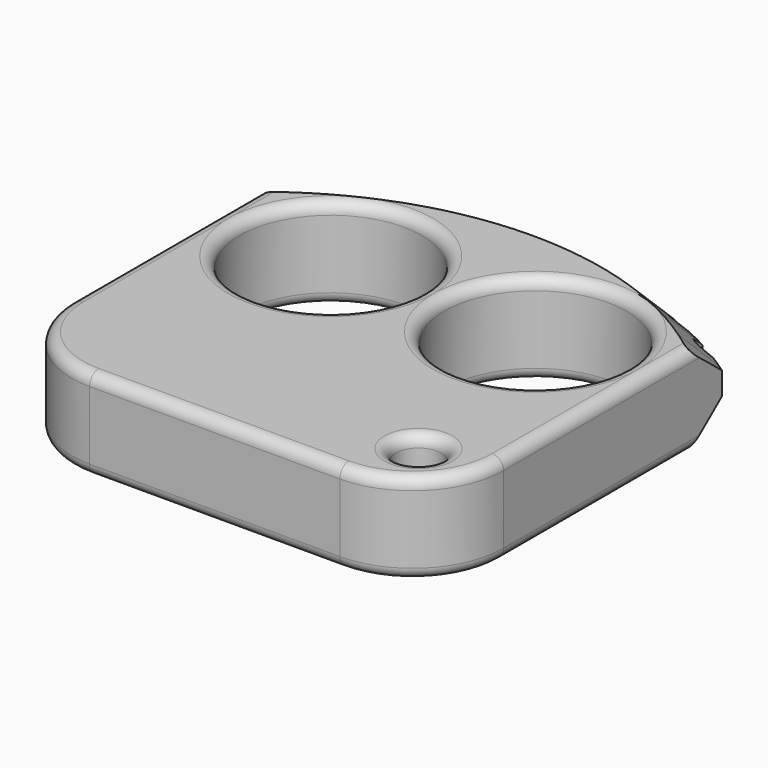
from build123d import *

# Parameters (mm, degrees)
F0_R         = 3.175
F0_R_2       = 12.7
F1_DEPTH     = 12.7
F2_R         = 1.58749
F3_T2_ANGLE  = 28.2217066526
F3_T4_ANGLE  = 30.4023138014
F3_T6_ANGLE  = 28.2217066526
F3_T8_ANGLE  = 30.7280198059
F3_T10_ANGLE = 30.527086938
F3_T12_ANGLE = 28.2217066526
F3_T14_ANGLE = 30.7280198059
F3_T16_ANGLE = 31.8182338751
F3_T18_ANGLE = 30.3249155811
F3_T20_ANGLE = 32.0978046052
F3_T22_ANGLE = 30.3249155811
F3_T24_ANGLE = 30.7280198059
F3_T26_ANGLE = 30.527086938
F3_T28_ANGLE = 28.2217066526
F3_T30_ANGLE = 30.4023138014
F3_T32_ANGLE = 30.7280198059
F3_T34_ANGLE = 31.8182338751
F3_T36_ANGLE = 30.3249155811
F3_T38_ANGLE = 32.0978046052
F3_T40_ANGLE = 30.3249155811
F4_DEPTH     = 25.4
F5_R         = 1.5875


# Not quite as in the source:
# - a fillet or chamfer that OpenCascade refuses, or shapes differently, is made with other operations: its cross-section is extruded or revolved along the edge and cut away or added
# - a fillet or chamfer is up to 0.001 mm smaller than in the source, because OpenCascade refuses the exact size


with BuildPart() as f1:
    # F0 (on Top) → F1 (new body)
    with BuildSketch(Plane.XY):
        with BuildLine():
            Line((30.1625, -25.4), (30.1625, 12.7))
            ThreePointArc((30.1625, 12.7), (28.8519314022, 13.5961848997), (27.5147547248, 14.4521615101))
            ThreePointArc((27.5147547248, 14.4521615101), (25.3582525776, 13.8924409049), (24.7658556955, 16.0401966174))
            ThreePointArc((24.7658556955, 16.0401966174), (23.1916703305, 16.8528451099), (21.5908556955, 17.6116926836))
            ThreePointArc((21.5908556955, 17.6116926836), (19.5238646988, 16.7802259757), (18.6611120255, 18.8343551079))
            ThreePointArc((18.6611120255, 18.8343551079), (17.1695789211, 19.3784749682), (15.6622115379, 19.8770539453))
            ThreePointArc((15.6622115379, 19.8770539453), (13.7112016409, 18.8012523611), (12.6059031197, 20.7357041816))
            ThreePointArc((12.6059031197, 20.7357041816), (11.059428231, 21.095082593), (9.5027540199, 21.4073370162))
            ThreePointArc((9.5027540199, 21.4073370162), (7.6964771744, 20.103054599), (6.3649215437, 21.8893211718))
            ThreePointArc((6.3649215437, 21.8893211718), (3.980300573, 22.1264782009), (1.5873170269, 22.2541119659))
            ThreePointArc((1.5873170269, 22.2541119659), (0, 20.6907139607), (-1.5873170269, 22.2541119659))
            ThreePointArc((-1.5873170269, 22.2541119659), (-3.8531098679, 22.1360337195), (-6.1116459836, 21.9197600851))
            ThreePointArc((-6.1116459836, 21.9197600851), (-7.4519015724, 20.1400118941), (-9.2517928734, 21.4530922311))
            ThreePointArc((-9.2517928734, 21.4530922311), (-10.8445183187, 21.1411241295), (-12.4267928734, 20.7798684392))
            ThreePointArc((-12.4267928734, 20.7798684392), (-13.5389102559, 18.8493287233), (-15.4861120255, 19.9320077778))
            ThreePointArc((-15.4861120255, 19.9320077778), (-17.0824306802, 19.4086897201), (-18.6611120255, 18.8343551079))
            ThreePointArc((-18.6611120255, 18.8343551079), (-19.5238646988, 16.7802259757), (-21.5908556955, 17.6116926836))
            ThreePointArc((-21.5908556955, 17.6116926836), (-23.1916703305, 16.8528451099), (-24.7658556955, 16.0401966174))
            ThreePointArc((-24.7658556955, 16.0401966174), (-25.3582525776, 13.8924409049), (-27.5147547248, 14.4521615101))
            ThreePointArc((-27.5147547248, 14.4521615101), (-28.8519314022, 13.5961848997), (-30.1625, 12.7))
            Line((-30.1625, 12.7), (-30.1625, -25.4))
            ThreePointArc((-30.1625, -25.4), (-26.4427561211, -34.3802561211), (-17.4625, -38.1))
            Line((-17.4625, -38.1), (17.4625, -38.1))
            ThreePointArc((17.4625, -38.1), (26.4427561211, -34.3802561211), (30.1625, -25.4))
        make_face()
        with Locations((21.5674359697, -29.5049359697)):
            Circle(F0_R, mode=Mode.SUBTRACT)
        with Locations((-14.2875, 0)):
            Circle(F0_R_2, mode=Mode.SUBTRACT)
        with Locations((14.2875, 0)):
            Circle(F0_R_2, mode=Mode.SUBTRACT)
    extrude(amount=F1_DEPTH)

    # F2 (radius 1.5875 in the source; OpenCascade refuses exactly that, so slightly less here)
    f2_edges = [f1.edges().sort_by_distance(p)[0] for p in [
        (0, -38.1, 12.7),
        (0, -38.1, 0),
        (-1.5875, 0, 6.35),
        (-26.9875, 0, 0),
        (-26.9875, 0, 12.7),
        (26.9875, 0, 6.35),
        (1.5875, 0, 0),
        (1.5875, 0, 12.7),
    ]]
    fillet(f2_edges, radius=F2_R)

    # F3: chamfer of 4.7625 on 20 edges, made by hand

    # F3_s1 → F3_t2 (revolve, cut)
    with BuildSketch(Plane(origin=(-8.957835853, -2.9681397895, 0), x_dir=(0, 0, 1), z_dir=(0.9492478243, 0.3145291211, 0))):
        Polygon((7.9375, -23.8009242864), (12.7, -19.0384242864), (12.7, -23.8009242864), align=None)
    revolve(axis=Axis((0, -30.0028581179, 12.7), (0, 0, 1)), revolution_arc=F3_T2_ANGLE, mode=Mode.SUBTRACT)

    # F3_s3 → F3_t4 (revolve, cut)
    with BuildSketch(Plane(origin=(1.6875607635, -0.0952218794, 0), x_dir=(0, 0, 1), z_dir=(0.9984118588, -0.0563361365, 0))):
        Polygon((0, -17.5633627369), (4.7625, -22.3258627369), (0, -22.3258627369), align=None)
    revolve(axis=Axis((0, -30.0028581179, 0), (0, 0, 1)), revolution_arc=F3_T4_ANGLE, mode=Mode.SUBTRACT)

    # F3_s5 → F3_t6 (revolve, cut)
    with BuildSketch(Plane(origin=(-8.957835853, -2.9681397895, 0), x_dir=(0, 0, 1), z_dir=(0.9492478243, 0.3145291211, 0))):
        Polygon((4.7625, -23.8009242864), (0, -19.0384242864), (0, -23.8009242864), align=None)
    revolve(axis=Axis((0, -30.0028581179, 0), (0, 0, 1)), revolution_arc=F3_T6_ANGLE, mode=Mode.SUBTRACT)

    # F3_s7 → F3_t8 (revolve, cut)
    with BuildSketch(Plane(origin=(-5.604837916, -1.0863772895, 0), x_dir=(0, 0, 1), z_dir=(0.9817285131, 0.1902869587, 0))):
        Polygon((0, -18.0639107911), (4.7625, -22.8264107911), (0, -22.8264107911), align=None)
    revolve(axis=Axis((0, -30.0028581179, 0), (0, 0, 1)), revolution_arc=F3_T8_ANGLE, mode=Mode.SUBTRACT)

    # F3_s9 → F3_t10 (revolve, cut)
    with BuildSketch(Plane(origin=(-1.9879865723, -0.1323072557, 0), x_dir=(0, 0, 1), z_dir=(0.9977926529, 0.0664064886, 0))):
        Polygon((0, -17.5819406812), (4.7625, -22.3444406812), (0, -22.3444406812), align=None)
    revolve(axis=Axis((0, -30.0028581179, 0), (0, 0, 1)), revolution_arc=F3_T10_ANGLE, mode=Mode.SUBTRACT)

    # F3_s11 → F3_t12 (revolve, cut)
    with BuildSketch(Plane(origin=(14.9793608703, -15.8148303911, 0), x_dir=(0, 0, 1), z_dir=(0.687669401, -0.726023963, 0))):
        Polygon((0, -26.8865246073), (4.7625, -31.6490246073), (0, -31.6490246073), align=None)
    revolve(axis=Axis((0, -30.0028581179, 0), (0, 0, 1)), revolution_arc=F3_T12_ANGLE, mode=Mode.SUBTRACT)

    # F3_s13 → F3_t14 (revolve, cut)
    with BuildSketch(Plane(origin=(14.9018636239, -13.275933668, 0), x_dir=(0, 0, 1), z_dir=(0.746666615, -0.6651984411, 0))):
        Polygon((0, -25.1164395681), (4.7625, -29.8789395681), (0, -29.8789395681), align=None)
    revolve(axis=Axis((0, -30.0028581179, 0), (0, 0, 1)), revolution_arc=F3_T14_ANGLE, mode=Mode.SUBTRACT)

    # F3_s15 → F3_t16 (revolve, cut)
    with BuildSketch(Plane(origin=(5.9494186304, -1.2301803221, 0), x_dir=(0, 0, 1), z_dir=(0.9792843793, -0.2024897638, 0))):
        Polygon((0, -18.1372417891), (4.7625, -22.8997417891), (0, -22.8997417891), align=None)
    revolve(axis=Axis((0, -30.0028581179, 0), (0, 0, 1)), revolution_arc=F3_T16_ANGLE, mode=Mode.SUBTRACT)

    # F3_s17 → F3_t18 (revolve, cut)
    with BuildSketch(Plane(origin=(13.9737874605, -9.5446774776, 0), x_dir=(0, 0, 1), z_dir=(0.8257568602, -0.5640262475, 0))):
        Polygon((0, -22.7435061634), (4.7625, -27.5060061634), (0, -27.5060061634), align=None)
    revolve(axis=Axis((0, -30.0028581179, 0), (0, 0, 1)), revolution_arc=F3_T18_ANGLE, mode=Mode.SUBTRACT)

    # F3_s19 → F3_t20 (revolve, cut)
    with BuildSketch(Plane(origin=(9.808271153, -3.6506277304, 0), x_dir=(0, 0, 1), z_dir=(0.9371894158, -0.3488208693, 0))):
        Polygon((0, -19.4002110061), (4.7625, -24.1627110061), (0, -24.1627110061), align=None)
    revolve(axis=Axis((0, -30.0028581179, 0), (0, 0, 1)), revolution_arc=F3_T20_ANGLE, mode=Mode.SUBTRACT)

    # F3_s21 → F3_t22 (revolve, cut)
    with BuildSketch(Plane(origin=(12.2507752992, -6.3434051286, 0), x_dir=(0, 0, 1), z_dir=(0.8880165005, -0.4598115863, 0))):
        Polygon((0, -20.8755390083), (4.7625, -25.6380390083), (0, -25.6380390083), align=None)
    revolve(axis=Axis((0, -30.0028581179, 0), (0, 0, 1)), revolution_arc=F3_T22_ANGLE, mode=Mode.SUBTRACT)

    # F3_s23 → F3_t24 (revolve, cut)
    with BuildSketch(Plane(origin=(-5.604837916, -1.0863772895, 0), x_dir=(0, 0, 1), z_dir=(0.9817285131, 0.1902869587, 0))):
        Polygon((12.7, -18.0639107911), (7.9375, -22.8264107911), (12.7, -22.8264107911), align=None)
    revolve(axis=Axis((0, -30.0028581179, 12.7), (0, 0, 1)), revolution_arc=F3_T24_ANGLE, mode=Mode.SUBTRACT)

    # F3_s25 → F3_t26 (revolve, cut)
    with BuildSketch(Plane(origin=(-1.9879865723, -0.1323072557, 0), x_dir=(0, 0, 1), z_dir=(0.9977926529, 0.0664064886, 0))):
        Polygon((12.7, -17.5819406812), (7.9375, -22.3444406812), (12.7, -22.3444406812), align=None)
    revolve(axis=Axis((0, -30.0028581179, 12.7), (0, 0, 1)), revolution_arc=F3_T26_ANGLE, mode=Mode.SUBTRACT)

    # F3_s27 → F3_t28 (revolve, cut)
    with BuildSketch(Plane(origin=(14.9793608703, -15.8148303911, 0), x_dir=(0, 0, 1), z_dir=(0.687669401, -0.726023963, 0))):
        Polygon((12.7, -26.8865246073), (7.9375, -31.6490246073), (12.7, -31.6490246073), align=None)
    revolve(axis=Axis((0, -30.0028581179, 12.7), (0, 0, 1)), revolution_arc=F3_T28_ANGLE, mode=Mode.SUBTRACT)

    # F3_s29 → F3_t30 (revolve, cut)
    with BuildSketch(Plane(origin=(1.6875607635, -0.0952218794, 0), x_dir=(0, 0, 1), z_dir=(0.9984118588, -0.0563361365, 0))):
        Polygon((12.7, -17.5633627369), (7.9375, -22.3258627369), (12.7, -22.3258627369), align=None)
    revolve(axis=Axis((0, -30.0028581179, 12.7), (0, 0, 1)), revolution_arc=F3_T30_ANGLE, mode=Mode.SUBTRACT)

    # F3_s31 → F3_t32 (revolve, cut)
    with BuildSketch(Plane(origin=(14.9018636239, -13.275933668, 0), x_dir=(0, 0, 1), z_dir=(0.746666615, -0.6651984411, 0))):
        Polygon((12.7, -25.1164395681), (7.9375, -29.8789395681), (12.7, -29.8789395681), align=None)
    revolve(axis=Axis((0, -30.0028581179, 12.7), (0, 0, 1)), revolution_arc=F3_T32_ANGLE, mode=Mode.SUBTRACT)

    # F3_s33 → F3_t34 (revolve, cut)
    with BuildSketch(Plane(origin=(5.9494186304, -1.2301803221, 0), x_dir=(0, 0, 1), z_dir=(0.9792843793, -0.2024897638, 0))):
        Polygon((12.7, -18.1372417891), (7.9375, -22.8997417891), (12.7, -22.8997417891), align=None)
    revolve(axis=Axis((0, -30.0028581179, 12.7), (0, 0, 1)), revolution_arc=F3_T34_ANGLE, mode=Mode.SUBTRACT)

    # F3_s35 → F3_t36 (revolve, cut)
    with BuildSketch(Plane(origin=(13.9737874605, -9.5446774776, 0), x_dir=(0, 0, 1), z_dir=(0.8257568602, -0.5640262475, 0))):
        Polygon((12.7, -22.7435061634), (7.9375, -27.5060061634), (12.7, -27.5060061634), align=None)
    revolve(axis=Axis((0, -30.0028581179, 12.7), (0, 0, 1)), revolution_arc=F3_T36_ANGLE, mode=Mode.SUBTRACT)

    # F3_s37 → F3_t38 (revolve, cut)
    with BuildSketch(Plane(origin=(9.808271153, -3.6506277304, 0), x_dir=(0, 0, 1), z_dir=(0.9371894158, -0.3488208693, 0))):
        Polygon((12.7, -19.4002110061), (7.9375, -24.1627110061), (12.7, -24.1627110061), align=None)
    revolve(axis=Axis((0, -30.0028581179, 12.7), (0, 0, 1)), revolution_arc=F3_T38_ANGLE, mode=Mode.SUBTRACT)

    # F3_s39 → F3_t40 (revolve, cut)
    with BuildSketch(Plane(origin=(12.2507752992, -6.3434051286, 0), x_dir=(0, 0, 1), z_dir=(0.8880165005, -0.4598115863, 0))):
        Polygon((12.7, -20.8755390083), (7.9375, -25.6380390083), (12.7, -25.6380390083), align=None)
    revolve(axis=Axis((0, -30.0028581179, 12.7), (0, 0, 1)), revolution_arc=F3_T40_ANGLE, mode=Mode.SUBTRACT)

    # F0 (on Top) → F4 (cut)
    with BuildSketch(Plane.XY):
        with Locations((21.5674359697, -29.5049359697)):
            Circle(F0_R)
    extrude(amount=F4_DEPTH, mode=Mode.SUBTRACT)

    # F5
    f5_edges = [f1.edges().sort_by_distance(p)[0] for p in [
        (24.742436, -29.504936, 6.35),
        (18.392436, -29.504936, 0),
        (18.392436, -29.504936, 12.7),
    ]]
    fillet(f5_edges, radius=F5_R)


solid = f1.part
